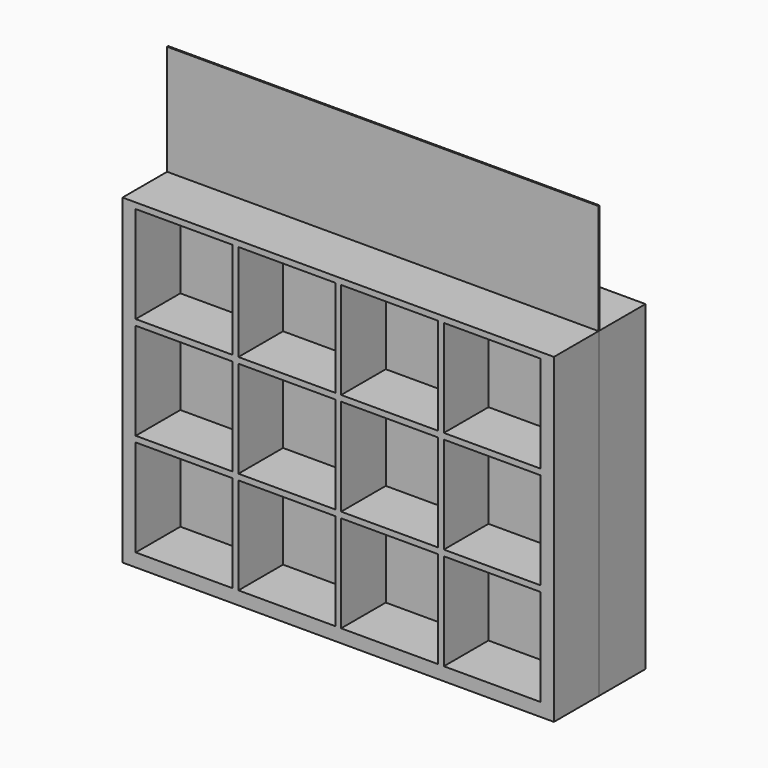
from build123d import *

# Parameters (mm, degrees)
F0_W     = 1470
F0_H     = 1470
F0_W_2   = 330
F0_H_2   = 330
F1_DEPTH = 195
F2_DEPTH = 5
F3_DEPTH = 375


with BuildPart() as f1:
    # F0 (on Front) → F1 (new body, symmetric)
    with BuildSketch(Plane.XZ):
        Rectangle(F0_W, F0_H)
        with Locations((-525, -525)):
            Rectangle(F0_W_2, F0_H_2, mode=Mode.SUBTRACT)
        with Locations((-175, -525)):
            Rectangle(F0_W_2, F0_H_2, mode=Mode.SUBTRACT)
        with Locations((-525, -175)):
            Rectangle(F0_W_2, F0_H_2, mode=Mode.SUBTRACT)
        with Locations((-175, -175)):
            Rectangle(F0_W_2, F0_H_2, mode=Mode.SUBTRACT)
        with Locations((175, -525)):
            Rectangle(F0_W_2, F0_H_2, mode=Mode.SUBTRACT)
        with Locations((525, -525)):
            Rectangle(F0_W_2, F0_H_2, mode=Mode.SUBTRACT)
        with Locations((175, -175)):
            Rectangle(F0_W_2, F0_H_2, mode=Mode.SUBTRACT)
        with Locations((525, -175)):
            Rectangle(F0_W_2, F0_H_2, mode=Mode.SUBTRACT)
        with Locations((-525, 175)):
            Rectangle(F0_W_2, F0_H_2, mode=Mode.SUBTRACT)
        with Locations((-175, 175)):
            Rectangle(F0_W_2, F0_H_2, mode=Mode.SUBTRACT)
        with Locations((-525, 525)):
            Rectangle(F0_W_2, F0_H_2, mode=Mode.SUBTRACT)
        with Locations((-175, 525)):
            Rectangle(F0_W_2, F0_H_2, mode=Mode.SUBTRACT)
        with Locations((175, 175)):
            Rectangle(F0_W_2, F0_H_2, mode=Mode.SUBTRACT)
        with Locations((525, 175)):
            Rectangle(F0_W_2, F0_H_2, mode=Mode.SUBTRACT)
        with Locations((175, 525)):
            Rectangle(F0_W_2, F0_H_2, mode=Mode.SUBTRACT)
        with Locations((525, 525)):
            Rectangle(F0_W_2, F0_H_2, mode=Mode.SUBTRACT)
    extrude(amount=F1_DEPTH, both=True)

    # F3 (cut, through all): a face of the model
    f3_faces = [f1.faces().sort_by_distance(p)[0] for p in [
        (0, 0, 735),
    ]]
    extrude(f3_faces, amount=-F3_DEPTH, mode=Mode.SUBTRACT)


with BuildPart() as f2:
    # F0 (on Front) → F2 (new body)
    with BuildSketch(Plane.XZ):
        Rectangle(F0_W, F0_H)
        with Locations((-525, -525)):
            Rectangle(F0_W_2, F0_H_2, mode=Mode.SUBTRACT)
        with Locations((-175, -525)):
            Rectangle(F0_W_2, F0_H_2, mode=Mode.SUBTRACT)
        with Locations((-525, -175)):
            Rectangle(F0_W_2, F0_H_2, mode=Mode.SUBTRACT)
        with Locations((-175, -175)):
            Rectangle(F0_W_2, F0_H_2, mode=Mode.SUBTRACT)
        with Locations((175, -525)):
            Rectangle(F0_W_2, F0_H_2, mode=Mode.SUBTRACT)
        with Locations((525, -525)):
            Rectangle(F0_W_2, F0_H_2, mode=Mode.SUBTRACT)
        with Locations((175, -175)):
            Rectangle(F0_W_2, F0_H_2, mode=Mode.SUBTRACT)
        with Locations((525, -175)):
            Rectangle(F0_W_2, F0_H_2, mode=Mode.SUBTRACT)
        with Locations((-525, 175)):
            Rectangle(F0_W_2, F0_H_2, mode=Mode.SUBTRACT)
        with Locations((-175, 175)):
            Rectangle(F0_W_2, F0_H_2, mode=Mode.SUBTRACT)
        with Locations((-525, 525)):
            Rectangle(F0_W_2, F0_H_2, mode=Mode.SUBTRACT)
        with Locations((-175, 525)):
            Rectangle(F0_W_2, F0_H_2, mode=Mode.SUBTRACT)
        with Locations((175, 175)):
            Rectangle(F0_W_2, F0_H_2, mode=Mode.SUBTRACT)
        with Locations((525, 175)):
            Rectangle(F0_W_2, F0_H_2, mode=Mode.SUBTRACT)
        with Locations((175, 525)):
            Rectangle(F0_W_2, F0_H_2, mode=Mode.SUBTRACT)
        with Locations((525, 525)):
            Rectangle(F0_W_2, F0_H_2, mode=Mode.SUBTRACT)
        with Locations((525, 525)):
            Rectangle(F0_W_2, F0_H_2)
        with Locations((175, 525)):
            Rectangle(F0_W_2, F0_H_2)
        with Locations((-175, 525)):
            Rectangle(F0_W_2, F0_H_2)
        with Locations((-525, 525)):
            Rectangle(F0_W_2, F0_H_2)
        with Locations((-525, 175)):
            Rectangle(F0_W_2, F0_H_2)
        with Locations((-175, 175)):
            Rectangle(F0_W_2, F0_H_2)
        with Locations((-175, -175)):
            Rectangle(F0_W_2, F0_H_2)
        with Locations((-525, -175)):
            Rectangle(F0_W_2, F0_H_2)
        with Locations((-525, -525)):
            Rectangle(F0_W_2, F0_H_2)
        with Locations((-175, -525)):
            Rectangle(F0_W_2, F0_H_2)
        with Locations((175, -525)):
            Rectangle(F0_W_2, F0_H_2)
        with Locations((525, -525)):
            Rectangle(F0_W_2, F0_H_2)
        with Locations((525, -175)):
            Rectangle(F0_W_2, F0_H_2)
        with Locations((525, 175)):
            Rectangle(F0_W_2, F0_H_2)
        with Locations((175, 175)):
            Rectangle(F0_W_2, F0_H_2)
        with Locations((175, -175)):
            Rectangle(F0_W_2, F0_H_2)
    extrude(amount=F2_DEPTH)


solid = Compound([f1.part, f2.part])
